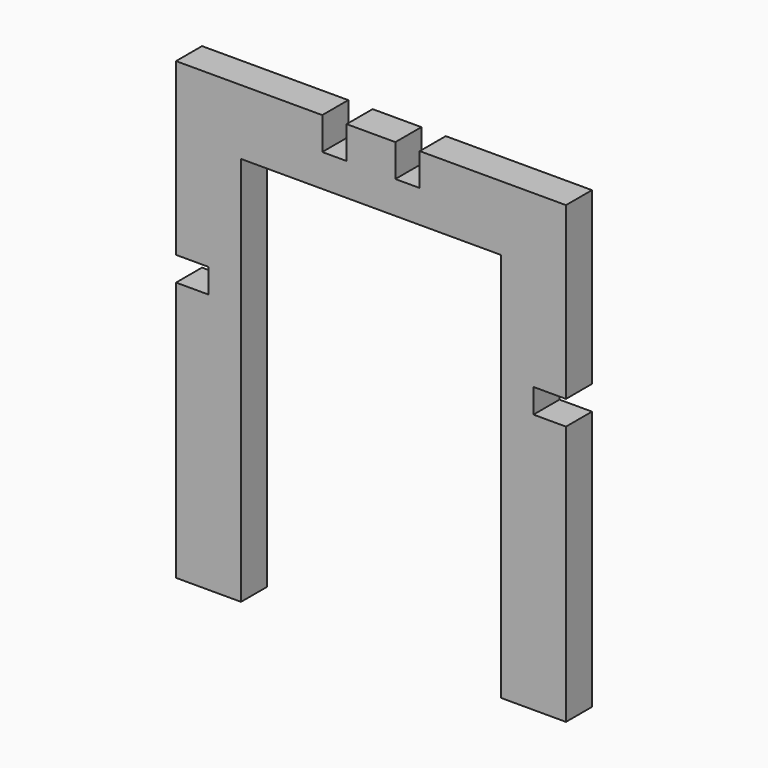
from build123d import *

# Parameters (mm, degrees)
F0_W     = 50.8
F0_H     = 50.8
F0_W_2   = 38.1
F0_H_2   = 25.4
F1_DEPTH = 25.4


# Not quite as in the source:
# - a feature names something its author has since deleted; it is built from what else it names


with BuildPart() as f1:
    # F0 (on Front) → F1 (new body)
    with BuildSketch(Plane.XZ):
        with Locations((-196.0164945363, -25.4)):
            Rectangle(F0_W, F0_H)
        with Locations((57.9835054637, -25.4)):
            Rectangle(F0_W, F0_H)
        Polygon((32.5835054637, -355.6), (83.3835054637, -355.6), (83.3835054637, -152.4), (57.9835054637, -152.4), (57.9835054637, -133.35), (83.3835054637, -133.35), (83.3835054637, -50.8), (32.5835054637, -50.8), align=None)
        Polygon((-170.6164945363, -355.6), (-170.6164945363, -50.8), (-221.4164945363, -50.8), (-221.4164945363, -133.35), (-196.0164945363, -133.35), (-196.0164945363, -152.4), (-221.4164945363, -152.4), (-221.4164945363, -355.6), align=None)
        Polygon((-170.6164945363, -50.8), (32.5835054637, -50.8), (32.5835054637, 0), (-30.9164945363, 0), (-30.9164945363, -25.4), (-49.9664945363, -25.4), (-88.0664945363, -25.4), (-107.1164945363, -25.4), (-107.1164945363, 0), (-170.6164945363, 0), align=None)
        with Locations((-69.0164945363, -12.7)):
            Rectangle(F0_W_2, F0_H_2)
    extrude(amount=F1_DEPTH)


solid = f1.part
